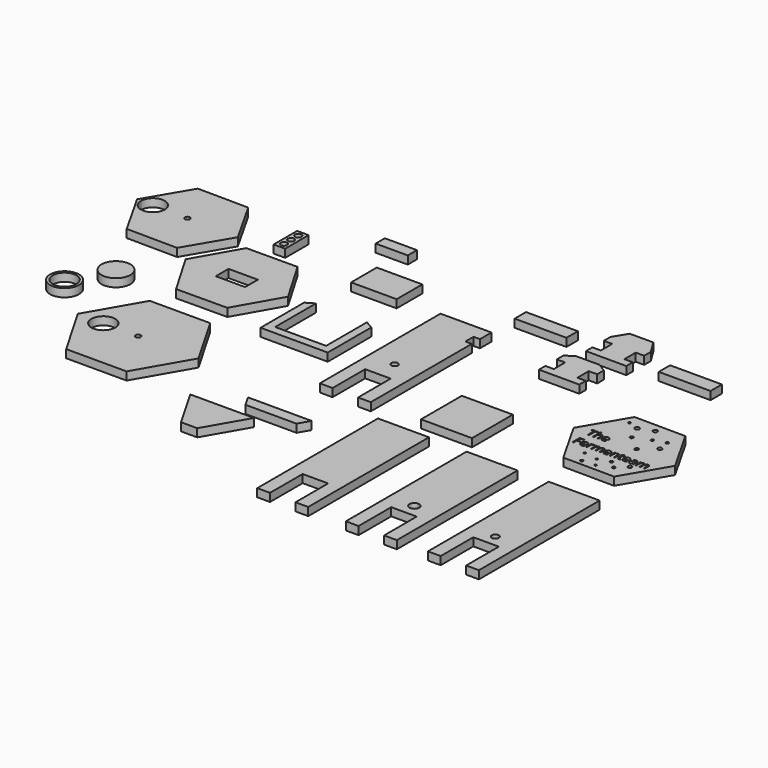
from build123d import *

# Parameters (mm, degrees)
F0_W     = 23
F0_H     = 12.5
F1_DEPTH = 6.35
F0_R     = 11.32
F0_W_2   = 40.64
F0_H_2   = 11.1560076475
F0_W_3   = 5
F0_H_3   = 11.35
F0_R_2   = 9.32
F0_R_3   = 1.1414075771
F0_R_4   = 0.7749819398
F0_R_5   = 0.8220081557
F0_R_6   = 0.8376599841
F0_R_7   = 1.1188046282
F0_R_8   = 1.1999997968
F0_R_9   = 1.5179013783
F0_R_10  = 1.4137050081
F0_R_11  = 1.2987416609
F0_R_12  = 1.1020189368
F0_R_13  = 0.9293109179
F0_R_14  = 1.7424434423
F0_R_15  = 1.6632093964
F0_R_16  = 1.1616311967
F0_R_17  = 1.6631997695
F0_W_4   = 25.2
F0_H_4   = 9
F0_W_5   = 15
F0_H_5   = 40
F0_W_6   = 10
F0_W_7   = 35.7
F0_H_6   = 25.2


# Not quite as in the source:
# - a feature names something its author has since deleted; it is built from what else it names


with BuildPart() as f1:
    # F0 (on Top) → F1 (new body)
    with BuildSketch(Plane.XY):
        Polygon((-93.5948539071, 0.11056655), (-73.7855066292, 34.8609587841), (-93.9755554565, 69.3915528762), (-133.9749515616, 69.1717547342), (-153.7842988395, 34.4213625001), (-133.5942500122, -0.109231592), align=None)
        with Locations((-113.7849027343, 34.6411606421)):
            Rectangle(F0_W, F0_H, mode=Mode.SUBTRACT)
    extrude(amount=F1_DEPTH)


with BuildPart() as f1b:
    # F0 (on Top) → F1, piece 2 (new body)
    with BuildSketch(Plane.XY):
        with Locations((-178.4373819828, -2.9960221145)):
            Circle(F0_R)
    extrude(amount=F1_DEPTH)


with BuildPart() as f1c:
    # F0 (on Top) → F1, piece 3 (new body)
    with BuildSketch(Plane.XY):
        Polygon((-20.9351536468, -136.0760015618), (-8.2351536468, -136.0760015618), (10.4148463532, -103.7732540007), (-39.5851536468, -103.7732540007), align=None)
    extrude(amount=F1_DEPTH)


with BuildPart() as f1d:
    # F0 (on Top) → F1, piece 4 (new body)
    with BuildSketch(Plane.XY):
        Polygon((40.420912765, -84.742741209), (-9.579087235, -84.742741209), (-4.579087235, -93.4029952469), (35.420912765, -93.4029952469), align=None)
    extrude(amount=F1_DEPTH)


with BuildPart() as f1e:
    # F0 (on Top) → F1, piece 5 (new body)
    with BuildSketch(Plane.XY):
        Polygon((138.8155827246, 127.2342521906), (120.3497827246, 127.2342521906), (113.7457827246, 116.4570544124), (113.7457827246, 109.9662874103), (120.3497827246, 109.9662874103), (120.3497827246, 98.8102797627), (113.7457827246, 98.8102797627), (113.7457827246, 92.4602797627), (145.4195827246, 92.4602797627), (145.4195827246, 98.8102797627), (138.8155827246, 98.8102797627), (138.8155827246, 109.9662874103), (145.4195827246, 109.9662874103), (145.4195827246, 116.4570544124), align=None)
    extrude(amount=F1_DEPTH)


with BuildPart() as f1f:
    # F0 (on Top) → F1, piece 6 (new body)
    with BuildSketch(Plane.XY):
        with Locations((186.0756911215, 104.3882835865)):
            Rectangle(F0_W_2, F0_H_2)
    extrude(amount=F1_DEPTH)


with BuildPart() as f1g:
    # F0 (on Top) → F1, piece 7 (new body)
    with BuildSketch(Plane.XY):
        with Locations((73.0896743277, 104.3882835865)):
            Rectangle(F0_W_2, F0_H_2)
    extrude(amount=F1_DEPTH)


with BuildPart() as f1h:
    # F0 (on Top) → F1, piece 8 (new body)
    with BuildSketch(Plane.XY):
        with BuildLine():
            Line((33.1884920597, 75.6191478133), (13.1884920597, 75.6191478133))
            Line((13.1884920597, 75.6191478133), (13.1884920597, -42.7308521867))
            Line((13.1884920597, -42.7308521867), (23.1884920597, -42.7308521867))
            Line((23.1884920597, -42.7308521867), (23.1884920597, -10.7308521867))
            Line((23.1884920597, -10.7308521867), (33.1884920597, -10.7308521867))
            Line((33.1884920597, -10.7308521867), (33.1884920597, 3.0191478133))
            ThreePointArc((33.1884920597, 3.0191478133), (30.5884920597, 5.6191478133), (33.1884920597, 8.2191478133))
            Line((33.1884920597, 8.2191478133), (33.1884920597, 75.6191478133))
        make_face()
        with BuildLine():
            Line((48.1884920597, 75.6191478133), (33.1884920597, 75.6191478133))
            Line((33.1884920597, 75.6191478133), (33.1884920597, 8.2191478133))
            ThreePointArc((33.1884920597, 8.2191478133), (35.0269696908, 7.4576254444), (35.7884920597, 5.6191478133))
            ThreePointArc((35.7884920597, 5.6191478133), (35.0269696908, 3.7806701822), (33.1884920597, 3.0191478133))
            Line((33.1884920597, 3.0191478133), (33.1884920597, -10.7308521867))
            Line((33.1884920597, -10.7308521867), (43.1884920597, -10.7308521867))
            Line((43.1884920597, -10.7308521867), (43.1884920597, -42.7308521867))
            Line((43.1884920597, -42.7308521867), (53.1884920597, -42.7308521867))
            Line((53.1884920597, -42.7308521867), (53.1884920597, 56.2691478133))
            Line((53.1884920597, 56.2691478133), (48.1884920597, 56.2691478133))
            Line((48.1884920597, 56.2691478133), (48.1884920597, 64.2691478133))
            Line((48.1884920597, 64.2691478133), (48.1884920597, 75.6191478133))
        make_face()
        with Locations((50.6884920597, 69.9441478133)):
            Rectangle(F0_W_3, F0_H_3)
    extrude(amount=F1_DEPTH)


with BuildPart() as f1i:
    # F0 (on Top) → F1, piece 9 (new body)
    with BuildSketch(Plane.XY):
        with Locations((-194.700971096, -33.0629588499)):
            Circle(F0_R)
        with Locations((-194.700971096, -33.0629588499)):
            Circle(F0_R_2, mode=Mode.SUBTRACT)
    extrude(amount=F1_DEPTH)


with BuildPart() as f1j:
    # F0 (on Top) → F1, piece 10 (new body)
    with BuildSketch(Plane.XY):
        Polygon((-136.4517834177, -104.2957006316), (-89.1217834177, -104.2957006316), (-65.4567834177, -63.3067182704), (-89.1217834177, -22.3177359093), (-136.4517834177, -22.3177359093), (-160.1167834177, -63.3067182704), align=None)
        with BuildLine():
            ThreePointArc((-130.7867834177, -63.3067182704), (-140.1067834177, -72.6267182704), (-149.4267834177, -63.3067182704))
            ThreePointArc((-149.4267834177, -63.3067182704), (-140.1067834177, -53.9867182704), (-130.7867834177, -63.3067182704))
        make_face(mode=Mode.SUBTRACT)
        with BuildLine():
            ThreePointArc((-110.7867834177, -63.3067182704), (-112.7867834177, -65.3067182704), (-114.7867834177, -63.3067182704))
            ThreePointArc((-114.7867834177, -63.3067182704), (-112.7867834177, -61.3067182704), (-110.7867834177, -63.3067182704))
        make_face(mode=Mode.SUBTRACT)
    extrude(amount=F1_DEPTH)


with BuildPart() as f1k:
    # F0 (on Top) → F1, piece 11 (new body)
    with BuildSketch(Plane.XY):
        Polygon((-207.0955206407, 43.3388591181), (-167.2973292077, 42.9594402712), (-147.0696471311, 77.2359756534), (-166.6401564875, 111.8919298825), (-206.4383479205, 112.2713487294), (-226.6660299971, 77.9948133472), align=None)
        with BuildLine():
            ThreePointArc((-204.8670206192, 77.7869909637), (-214.2754459411, 68.5562633129), (-223.5061735919, 77.9646886347))
            ThreePointArc((-223.5061735919, 77.9646886347), (-214.1421721831, 87.1957339202), (-204.8665971055, 77.8758397992))
            ThreePointArc((-204.8665971055, 77.8758397992), (-204.8667029846, 77.8314148768), (-204.8670206192, 77.7869909637))
        make_face(mode=Mode.SUBTRACT)
        with BuildLine():
            ThreePointArc((-184.8678385641, 77.6153945003), (-186.8773718092, 75.6154172211), (-188.8677476813, 77.634460774))
            ThreePointArc((-188.8677476813, 77.634460774), (-186.8583053189, 79.6153717795), (-184.8678385641, 77.6153945003))
        make_face(mode=Mode.SUBTRACT)
    extrude(amount=F1_DEPTH)


with BuildPart() as f1l:
    # F0 (on Top) → F1, piece 12 (new body)
    with BuildSketch(Plane.XY):
        Polygon((251.4182813621, 7.740817484), (231.6635930538, 42.5234644066), (191.6635930538, 42.806725949), (171.4182813621, 8.3073405689), (191.1729696704, -26.4753063537), (231.1729696704, -26.7585678962), align=None)
        with Locations((202.5459110737, -22.6449556649)):
            Circle(F0_R_3, mode=Mode.SUBTRACT)
        with Locations((212.8806561232, -22.0124032348)):
            Circle(F0_R_4, mode=Mode.SUBTRACT)
        Polygon((183.5228956864, -3.8237476475), (183.5228956864, -6.7932858103), (182.7155097343, -6.7932858103), (182.7155097343, 0.1538825798), (186.5882254029, 0.1538825798), (186.5882254029, -0.563793822), (183.5228956864, -0.563793822), (183.5228956864, -3.1060712456), (186.402724299, -3.1060712456), (186.402724299, -3.8237476475), align=None, mode=Mode.SUBTRACT)
        with BuildLine():
            add(Edge.make_bspline(
                [(190.7194262162, -6.8100113196), (190.3469035076, -6.8890773639), (189.8192897122, -6.8890773639)],
                knots=[0, 0, 0, 1, 1, 1], degree=2))
            add(Edge.make_bspline(
                [(189.8192897122, -6.8890773639), (188.6652295659, -6.8890773639), (187.9969694417, -6.1850854697)],
                knots=[0, 0, 0, 1, 1, 1], degree=2))
            add(Edge.make_bspline(
                [(187.9969694417, -6.1850854697), (187.3287093175, -5.4810935755), (187.3287093175, -4.2327623765)],
                knots=[0, 0, 0, 1, 1, 1], degree=2))
            add(Edge.make_bspline(
                [(187.3287093175, -4.2327623765), (187.3287093175, -2.9722671707), (187.9490736649, -2.2310230056)],
                knots=[0, 0, 0, 1, 1, 1], degree=2))
            add(Edge.make_bspline(
                [(187.9490736649, -2.2310230056), (188.5694380123, -1.4897788405), (189.6155425981, -1.4897788405)],
                knots=[0, 0, 0, 1, 1, 1], degree=2))
            add(Edge.make_bspline(
                [(189.6155425981, -1.4897788405), (190.5932246455, -1.4897788405), (191.1634124648, -2.1337109511)],
                knots=[0, 0, 0, 1, 1, 1], degree=2))
            add(Edge.make_bspline(
                [(191.1634124648, -2.1337109511), (191.7336002841, -2.7776430617), (191.7336002841, -3.8328706526)],
                knots=[0, 0, 0, 1, 1, 1], degree=2))
            Line((191.7336002841, -3.8328706526), (191.7336002841, -4.3315949318))
            Line((191.7336002841, -4.3315949318), (188.1467387756, -4.3315949318))
            add(Edge.make_bspline(
                [(188.1467387756, -4.3315949318), (188.1710667892, -5.2484569452), (188.6104915353, -5.7236134613)],
                knots=[0, 0, 0, 1, 1, 1], degree=2))
            add(Edge.make_bspline(
                [(188.6104915353, -5.7236134613), (189.0499162813, -6.1987699774), (189.8481792283, -6.1987699774)],
                knots=[0, 0, 0, 1, 1, 1], degree=2))
            add(Edge.make_bspline(
                [(189.8481792283, -6.1987699774), (190.6890161992, -6.1987699774), (191.5100866589, -5.8475342807)],
                knots=[0, 0, 0, 1, 1, 1], degree=2))
            Line((191.5100866589, -5.8475342807), (191.5100866589, -6.5515261749))
            add(Edge.make_bspline(
                [(191.5100866589, -6.5515261749), (191.0919489248, -6.7309452754), (190.7194262162, -6.8100113196)],
                knots=[0, 0, 0, 1, 1, 1], degree=2))
        make_face(mode=Mode.SUBTRACT)
        Polygon((184.8533339314, 12.6706455887), (184.8533339314, 6.4411536005), (184.0459479793, 6.4411536005), (184.0459479793, 12.6706455887), (181.8457832473, 12.6706455887), (181.8457832473, 13.3883219906), (187.0534986634, 13.3883219906), (187.0534986634, 12.6706455887), align=None, mode=Mode.SUBTRACT)
        with BuildLine():
            Line((192.3341981204, 6.4411536005), (191.5450581785, 6.4411536005))
            Line((191.5450581785, 6.4411536005), (191.5450581785, 9.8105834872))
            add(Edge.make_bspline(
                [(191.5450581785, 9.8105834872), (191.5450581785, 10.4461528431), (191.2554027663, 10.7601362689)],
                knots=[0, 0, 0, 1, 1, 1], degree=2))
            add(Edge.make_bspline(
                [(191.2554027663, 10.7601362689), (190.9657473541, 11.0741196947), (190.3469035076, 11.0741196947)],
                knots=[0, 0, 0, 1, 1, 1], degree=2))
            add(Edge.make_bspline(
                [(190.3469035076, 11.0741196947), (189.5258330478, 11.0741196947), (189.1479885863, 10.6270924444)],
                knots=[0, 0, 0, 1, 1, 1], degree=2))
            add(Edge.make_bspline(
                [(189.1479885863, 10.6270924444), (188.7701441247, 10.1800651941), (188.7701441247, 9.1643706253)],
                knots=[0, 0, 0, 1, 1, 1], degree=2))
            Line((188.7701441247, 9.1643706253), (188.7701441247, 6.4411536005))
            Line((188.7701441247, 6.4411536005), (187.9810041828, 6.4411536005))
            Line((187.9810041828, 6.4411536005), (187.9810041828, 13.8353492409))
            Line((187.9810041828, 13.8353492409), (188.7701441247, 13.8353492409))
            Line((188.7701441247, 13.8353492409), (188.7701441247, 11.5971719876))
            add(Edge.make_bspline(
                [(188.7701441247, 11.5971719876), (188.7701441247, 11.1927187611), (188.7321316034, 10.9266311121)],
                knots=[0, 0, 0, 1, 1, 1], degree=2))
            Line((188.7321316034, 10.9266311121), (188.7792671298, 10.9266311121))
            add(Edge.make_bspline(
                [(188.7792671298, 10.9266311121), (189.01190376, 11.3021948224), (189.442205501, 11.5181059433)],
                knots=[0, 0, 0, 1, 1, 1], degree=2))
            add(Edge.make_bspline(
                [(189.442205501, 11.5181059433), (189.872507242, 11.7340170642), (190.4229285502, 11.7340170642)],
                knots=[0, 0, 0, 1, 1, 1], degree=2))
            add(Edge.make_bspline(
                [(190.4229285502, 11.7340170642), (191.3778030849, 11.7340170642), (191.8560006026, 11.2801475601)],
                knots=[0, 0, 0, 1, 1, 1], degree=2))
            add(Edge.make_bspline(
                [(191.8560006026, 11.2801475601), (192.3341981204, 10.8262780559), (192.3341981204, 9.8379525025)],
                knots=[0, 0, 0, 1, 1, 1], degree=2))
            Line((192.3341981204, 9.8379525025), (192.3341981204, 6.4411536005))
        make_face(mode=Mode.SUBTRACT)
        with Locations((197.5992619991, -13.4883988649)):
            Circle(F0_R_5, mode=Mode.SUBTRACT)
        with Locations((208.3211392164, -15.1996426284)):
            Circle(F0_R_6, mode=Mode.SUBTRACT)
        with Locations((217.7015841007, -12.4359205365)):
            Circle(F0_R_7, mode=Mode.SUBTRACT)
        with BuildLine():
            add(Edge.make_bspline(
                [(194.5571703652, -1.7657497451), (194.9661850942, -1.4897788405), (195.4557863684, -1.4897788405)],
                knots=[0, 0, 0, 1, 1, 1], degree=2))
            add(Edge.make_bspline(
                [(195.4557863684, -1.4897788405), (195.8024605625, -1.4897788405), (196.0776712166, -1.5475578729)],
                knots=[0, 0, 0, 1, 1, 1], degree=2))
            Line((196.0776712166, -1.5475578729), (195.9681951553, -2.2789187824))
            add(Edge.make_bspline(
                [(195.9681951553, -2.2789187824), (195.6458489748, -2.2074552424), (195.398007336, -2.2074552424)],
                knots=[0, 0, 0, 1, 1, 1], degree=2))
            add(Edge.make_bspline(
                [(195.398007336, -2.2074552424), (194.7654789818, -2.2074552424), (194.3169312306, -2.7206242798)],
                knots=[0, 0, 0, 1, 1, 1], degree=2))
            add(Edge.make_bspline(
                [(194.3169312306, -2.7206242798), (193.8683834795, -3.2337933171), (193.8683834795, -3.9986052454)],
                knots=[0, 0, 0, 1, 1, 1], degree=2))
            Line((193.8683834795, -3.9986052454), (193.8683834795, -6.7932858103))
            Line((193.8683834795, -6.7932858103), (193.0792435376, -6.7932858103))
            Line((193.0792435376, -6.7932858103), (193.0792435376, -1.5855703942))
            Line((193.0792435376, -1.5855703942), (193.730017902, -1.5855703942))
            Line((193.730017902, -1.5855703942), (193.8212479531, -2.549567934))
            Line((193.8212479531, -2.549567934), (193.8592604744, -2.549567934))
            add(Edge.make_bspline(
                [(193.8592604744, -2.549567934), (194.1481556361, -2.0417206496), (194.5571703652, -1.7657497451)],
                knots=[0, 0, 0, 1, 1, 1], degree=2))
        make_face(mode=Mode.SUBTRACT)
        with BuildLine():
            Line((204.4784384207, -6.7932858103), (203.6908189796, -6.7932858103))
            Line((203.6908189796, -6.7932858103), (203.6908189796, -3.4056099133))
            add(Edge.make_bspline(
                [(203.6908189796, -3.4056099133), (203.6908189796, -2.7822045642), (203.4247313306, -2.4712621401)],
                knots=[0, 0, 0, 1, 1, 1], degree=2))
            add(Edge.make_bspline(
                [(203.4247313306, -2.4712621401), (203.1586436816, -2.160319716), (202.5975788675, -2.160319716)],
                knots=[0, 0, 0, 1, 1, 1], degree=2))
            add(Edge.make_bspline(
                [(202.5975788675, -2.160319716), (201.8616564554, -2.160319716), (201.5096605083, -2.5830189527)],
                knots=[0, 0, 0, 1, 1, 1], degree=2))
            add(Edge.make_bspline(
                [(201.5096605083, -2.5830189527), (201.1576645612, -3.0057181894), (201.1576645612, -3.8845676815)],
                knots=[0, 0, 0, 1, 1, 1], degree=2))
            Line((201.1576645612, -3.8845676815), (201.1576645612, -6.7932858103))
            Line((201.1576645612, -6.7932858103), (200.3685246193, -6.7932858103))
            Line((200.3685246193, -6.7932858103), (200.3685246193, -3.4056099133))
            add(Edge.make_bspline(
                [(200.3685246193, -3.4056099133), (200.3685246193, -2.7822045642), (200.1024369703, -2.4712621401)],
                knots=[0, 0, 0, 1, 1, 1], degree=2))
            add(Edge.make_bspline(
                [(200.1024369703, -2.4712621401), (199.8363493213, -2.160319716), (199.2707230046, -2.160319716)],
                knots=[0, 0, 0, 1, 1, 1], degree=2))
            add(Edge.make_bspline(
                [(199.2707230046, -2.160319716), (198.5302390899, -2.160319716), (198.1858456471, -2.6043059646)],
                knots=[0, 0, 0, 1, 1, 1], degree=2))
            add(Edge.make_bspline(
                [(198.1858456471, -2.6043059646), (197.8414522042, -3.0482922132), (197.8414522042, -4.0609457803)],
                knots=[0, 0, 0, 1, 1, 1], degree=2))
            Line((197.8414522042, -4.0609457803), (197.8414522042, -6.7932858103))
            Line((197.8414522042, -6.7932858103), (197.0523122623, -6.7932858103))
            Line((197.0523122623, -6.7932858103), (197.0523122623, -1.5855703942))
            Line((197.0523122623, -1.5855703942), (197.6939636216, -1.5855703942))
            Line((197.6939636216, -1.5855703942), (197.8216856932, -2.2986852935))
            Line((197.8216856932, -2.2986852935), (197.8596982144, -2.2986852935))
            add(Edge.make_bspline(
                [(197.8596982144, -2.2986852935), (198.0832118396, -1.9185600806), (198.4899458174, -1.7041694606)],
                knots=[0, 0, 0, 1, 1, 1], degree=2))
            add(Edge.make_bspline(
                [(198.4899458174, -1.7041694606), (198.8966797951, -1.4897788405), (199.3999655769, -1.4897788405)],
                knots=[0, 0, 0, 1, 1, 1], degree=2))
            add(Edge.make_bspline(
                [(199.3999655769, -1.4897788405), (200.6209277606, -1.4897788405), (200.9964914709, -2.3747103361)],
                knots=[0, 0, 0, 1, 1, 1], degree=2))
            Line((200.9964914709, -2.3747103361), (201.0345039922, -2.3747103361))
            add(Edge.make_bspline(
                [(201.0345039922, -2.3747103361), (201.2671406225, -1.965695607), (201.7088461198, -1.7277372238)],
                knots=[0, 0, 0, 1, 1, 1], degree=2))
            add(Edge.make_bspline(
                [(201.7088461198, -1.7277372238), (202.1505516171, -1.4897788405), (202.7161779339, -1.4897788405)],
                knots=[0, 0, 0, 1, 1, 1], degree=2))
            add(Edge.make_bspline(
                [(202.7161779339, -1.4897788405), (203.5995889285, -1.4897788405), (204.0390136746, -1.9436483447)],
                knots=[0, 0, 0, 1, 1, 1], degree=2))
            add(Edge.make_bspline(
                [(204.0390136746, -1.9436483447), (204.4784384207, -2.3975178488), (204.4784384207, -3.3964869082)],
                knots=[0, 0, 0, 1, 1, 1], degree=2))
            Line((204.4784384207, -3.3964869082), (204.4784384207, -6.7932858103))
        make_face(mode=Mode.SUBTRACT)
        with BuildLine():
            add(Edge.make_bspline(
                [(209.2041550669, -6.8100113196), (208.8316323583, -6.8890773639), (208.3040185628, -6.8890773639)],
                knots=[0, 0, 0, 1, 1, 1], degree=2))
            add(Edge.make_bspline(
                [(208.3040185628, -6.8890773639), (207.1499584166, -6.8890773639), (206.4816982924, -6.1850854697)],
                knots=[0, 0, 0, 1, 1, 1], degree=2))
            add(Edge.make_bspline(
                [(206.4816982924, -6.1850854697), (205.8134381682, -5.4810935755), (205.8134381682, -4.2327623765)],
                knots=[0, 0, 0, 1, 1, 1], degree=2))
            add(Edge.make_bspline(
                [(205.8134381682, -4.2327623765), (205.8134381682, -2.9722671707), (206.4338025156, -2.2310230056)],
                knots=[0, 0, 0, 1, 1, 1], degree=2))
            add(Edge.make_bspline(
                [(206.4338025156, -2.2310230056), (207.054166863, -1.4897788405), (208.1002714487, -1.4897788405)],
                knots=[0, 0, 0, 1, 1, 1], degree=2))
            add(Edge.make_bspline(
                [(208.1002714487, -1.4897788405), (209.0779534962, -1.4897788405), (209.6481413155, -2.1337109511)],
                knots=[0, 0, 0, 1, 1, 1], degree=2))
            add(Edge.make_bspline(
                [(209.6481413155, -2.1337109511), (210.2183291348, -2.7776430617), (210.2183291348, -3.8328706526)],
                knots=[0, 0, 0, 1, 1, 1], degree=2))
            Line((210.2183291348, -3.8328706526), (210.2183291348, -4.3315949318))
            Line((210.2183291348, -4.3315949318), (206.6314676263, -4.3315949318))
            add(Edge.make_bspline(
                [(206.6314676263, -4.3315949318), (206.6557956399, -5.2484569452), (207.095220386, -5.7236134613)],
                knots=[0, 0, 0, 1, 1, 1], degree=2))
            add(Edge.make_bspline(
                [(207.095220386, -5.7236134613), (207.534645132, -6.1987699774), (208.332908079, -6.1987699774)],
                knots=[0, 0, 0, 1, 1, 1], degree=2))
            add(Edge.make_bspline(
                [(208.332908079, -6.1987699774), (209.1737450498, -6.1987699774), (209.9948155096, -5.8475342807)],
                knots=[0, 0, 0, 1, 1, 1], degree=2))
            Line((209.9948155096, -5.8475342807), (209.9948155096, -6.5515261749))
            add(Edge.make_bspline(
                [(209.9948155096, -6.5515261749), (209.5766777755, -6.7309452754), (209.2041550669, -6.8100113196)],
                knots=[0, 0, 0, 1, 1, 1], degree=2))
        make_face(mode=Mode.SUBTRACT)
        with BuildLine():
            Line((215.9171663259, -6.7932858103), (215.128026384, -6.7932858103))
            Line((215.128026384, -6.7932858103), (215.128026384, -3.4238559235))
            add(Edge.make_bspline(
                [(215.128026384, -3.4238559235), (215.128026384, -2.7882865676), (214.8383709718, -2.4743031418)],
                knots=[0, 0, 0, 1, 1, 1], degree=2))
            add(Edge.make_bspline(
                [(214.8383709718, -2.4743031418), (214.5487155596, -2.160319716), (213.9298717131, -2.160319716)],
                knots=[0, 0, 0, 1, 1, 1], degree=2))
            add(Edge.make_bspline(
                [(213.9298717131, -2.160319716), (213.1133627559, -2.160319716), (212.733237543, -2.6020252133)],
                knots=[0, 0, 0, 1, 1, 1], degree=2))
            add(Edge.make_bspline(
                [(212.733237543, -2.6020252133), (212.3531123302, -3.0437307107), (212.3531123302, -4.0609457803)],
                knots=[0, 0, 0, 1, 1, 1], degree=2))
            Line((212.3531123302, -4.0609457803), (212.3531123302, -6.7932858103))
            Line((212.3531123302, -6.7932858103), (211.5639723883, -6.7932858103))
            Line((211.5639723883, -6.7932858103), (211.5639723883, -1.5855703942))
            Line((211.5639723883, -1.5855703942), (212.2056237476, -1.5855703942))
            Line((212.2056237476, -1.5855703942), (212.3333458191, -2.2986852935))
            Line((212.3333458191, -2.2986852935), (212.3713583404, -2.2986852935))
            add(Edge.make_bspline(
                [(212.3713583404, -2.2986852935), (212.6146384766, -1.9139985781), (213.0517824714, -1.7018887093)],
                knots=[0, 0, 0, 1, 1, 1], degree=2))
            add(Edge.make_bspline(
                [(213.0517824714, -1.7018887093), (213.4889264662, -1.4897788405), (214.0256632667, -1.4897788405)],
                knots=[0, 0, 0, 1, 1, 1], degree=2))
            add(Edge.make_bspline(
                [(214.0256632667, -1.4897788405), (214.9668532937, -1.4897788405), (215.4420098098, -1.9436483447)],
                knots=[0, 0, 0, 1, 1, 1], degree=2))
            add(Edge.make_bspline(
                [(215.4420098098, -1.9436483447), (215.9171663259, -2.3975178488), (215.9171663259, -3.3964869082)],
                knots=[0, 0, 0, 1, 1, 1], degree=2))
            Line((215.9171663259, -3.3964869082), (215.9171663259, -6.7932858103))
        make_face(mode=Mode.SUBTRACT)
        with BuildLine():
            add(Edge.make_bspline(
                [(218.6054118312, -5.9851396078), (218.8289254563, -6.2367824987), (219.2181736743, -6.2367824987)],
                knots=[0, 0, 0, 1, 1, 1], degree=2))
            add(Edge.make_bspline(
                [(219.2181736743, -6.2367824987), (219.4280027918, -6.2367824987), (219.6226269008, -6.2063724816)],
                knots=[0, 0, 0, 1, 1, 1], degree=2))
            add(Edge.make_bspline(
                [(219.6226269008, -6.2063724816), (219.8172510098, -6.1759624646), (219.9312885736, -6.1425114459)],
                knots=[0, 0, 0, 1, 1, 1], degree=2))
            Line((219.9312885736, -6.1425114459), (219.9312885736, -6.7461502839))
            add(Edge.make_bspline(
                [(219.9312885736, -6.7461502839), (219.8035665021, -6.8069703179), (219.5542043625, -6.8480238409)],
                knots=[0, 0, 0, 1, 1, 1], degree=2))
            add(Edge.make_bspline(
                [(219.5542043625, -6.8480238409), (219.3048422228, -6.8890773639), (219.1041361105, -6.8890773639)],
                knots=[0, 0, 0, 1, 1, 1], degree=2))
            add(Edge.make_bspline(
                [(219.1041361105, -6.8890773639), (217.594278765, -6.8890773639), (217.594278765, -5.2971129725)],
                knots=[0, 0, 0, 1, 1, 1], degree=2))
            Line((217.594278765, -5.2971129725), (217.594278765, -2.1983322373))
            Line((217.594278765, -2.1983322373), (216.847712847, -2.1983322373))
            Line((216.847712847, -2.1983322373), (216.847712847, -1.8182070244))
            Line((216.847712847, -1.8182070244), (217.594278765, -1.4897788405))
            Line((217.594278765, -1.4897788405), (217.9257479506, -0.3782927181))
            Line((217.9257479506, -0.3782927181), (218.381898206, -0.3782927181))
            Line((218.381898206, -0.3782927181), (218.381898206, -1.5855703942))
            Line((218.381898206, -1.5855703942), (219.8932760523, -1.5855703942))
            Line((219.8932760523, -1.5855703942), (219.8932760523, -2.1983322373))
            Line((219.8932760523, -2.1983322373), (218.381898206, -2.1983322373))
            Line((218.381898206, -2.1983322373), (218.381898206, -5.2636619538))
            add(Edge.make_bspline(
                [(218.381898206, -5.2636619538), (218.381898206, -5.7334967168), (218.6054118312, -5.9851396078)],
                knots=[0, 0, 0, 1, 1, 1], degree=2))
        make_face(mode=Mode.SUBTRACT)
        with Locations((223.384976387, -17.3825658858)):
            Circle(F0_R_8, mode=Mode.SUBTRACT)
        with Locations((230.6536883116, -10.4995090514)):
            Circle(F0_R_9, mode=Mode.SUBTRACT)
        with BuildLine():
            add(Edge.make_bspline(
                [(224.071612392, -6.8100113196), (223.6990896834, -6.8890773639), (223.171475888, -6.8890773639)],
                knots=[0, 0, 0, 1, 1, 1], degree=2))
            add(Edge.make_bspline(
                [(223.171475888, -6.8890773639), (222.0174157418, -6.8890773639), (221.3491556176, -6.1850854697)],
                knots=[0, 0, 0, 1, 1, 1], degree=2))
            add(Edge.make_bspline(
                [(221.3491556176, -6.1850854697), (220.6808954934, -5.4810935755), (220.6808954934, -4.2327623765)],
                knots=[0, 0, 0, 1, 1, 1], degree=2))
            add(Edge.make_bspline(
                [(220.6808954934, -4.2327623765), (220.6808954934, -2.9722671707), (221.3012598408, -2.2310230056)],
                knots=[0, 0, 0, 1, 1, 1], degree=2))
            add(Edge.make_bspline(
                [(221.3012598408, -2.2310230056), (221.9216241881, -1.4897788405), (222.9677287739, -1.4897788405)],
                knots=[0, 0, 0, 1, 1, 1], degree=2))
            add(Edge.make_bspline(
                [(222.9677287739, -1.4897788405), (223.9454108214, -1.4897788405), (224.5155986407, -2.1337109511)],
                knots=[0, 0, 0, 1, 1, 1], degree=2))
            add(Edge.make_bspline(
                [(224.5155986407, -2.1337109511), (225.0857864599, -2.7776430617), (225.0857864599, -3.8328706526)],
                knots=[0, 0, 0, 1, 1, 1], degree=2))
            Line((225.0857864599, -3.8328706526), (225.0857864599, -4.3315949318))
            Line((225.0857864599, -4.3315949318), (221.4989249514, -4.3315949318))
            add(Edge.make_bspline(
                [(221.4989249514, -4.3315949318), (221.5232529651, -5.2484569452), (221.9626777111, -5.7236134613)],
                knots=[0, 0, 0, 1, 1, 1], degree=2))
            add(Edge.make_bspline(
                [(221.9626777111, -5.7236134613), (222.4021024572, -6.1987699774), (223.2003654042, -6.1987699774)],
                knots=[0, 0, 0, 1, 1, 1], degree=2))
            add(Edge.make_bspline(
                [(223.2003654042, -6.1987699774), (224.041202375, -6.1987699774), (224.8622728348, -5.8475342807)],
                knots=[0, 0, 0, 1, 1, 1], degree=2))
            Line((224.8622728348, -5.8475342807), (224.8622728348, -6.5515261749))
            add(Edge.make_bspline(
                [(224.8622728348, -6.5515261749), (224.4441351006, -6.7309452754), (224.071612392, -6.8100113196)],
                knots=[0, 0, 0, 1, 1, 1], degree=2))
        make_face(mode=Mode.SUBTRACT)
        with BuildLine():
            Line((230.2189973343, -6.7932858103), (229.6336045065, -6.7932858103))
            Line((229.6336045065, -6.7932858103), (229.4769929188, -6.0512813948))
            Line((229.4769929188, -6.0512813948), (229.4389803975, -6.0512813948))
            add(Edge.make_bspline(
                [(229.4389803975, -6.0512813948), (229.0497321796, -6.5408826689), (228.6627647129, -6.7149800164)],
                knots=[0, 0, 0, 1, 1, 1], degree=2))
            add(Edge.make_bspline(
                [(228.6627647129, -6.7149800164), (228.2757972462, -6.8890773639), (227.694965921, -6.8890773639)],
                knots=[0, 0, 0, 1, 1, 1], degree=2))
            add(Edge.make_bspline(
                [(227.694965921, -6.8890773639), (226.9210309876, -6.8890773639), (226.4816062415, -6.48918564)],
                knots=[0, 0, 0, 1, 1, 1], degree=2))
            add(Edge.make_bspline(
                [(226.4816062415, -6.48918564), (226.0421814955, -6.0892939161), (226.0421814955, -5.353371504)],
                knots=[0, 0, 0, 1, 1, 1], degree=2))
            add(Edge.make_bspline(
                [(226.0421814955, -5.353371504), (226.0421814955, -3.7766121211), (228.564692408, -3.7005870785)],
                knots=[0, 0, 0, 1, 1, 1], degree=2))
            Line((228.564692408, -3.7005870785), (229.4481034026, -3.6716975623))
            Line((229.4481034026, -3.6716975623), (229.4481034026, -3.347830881))
            add(Edge.make_bspline(
                [(229.4481034026, -3.347830881), (229.4481034026, -2.7350690378), (229.1850567554, -2.4431328744)],
                knots=[0, 0, 0, 1, 1, 1], degree=2))
            add(Edge.make_bspline(
                [(229.1850567554, -2.4431328744), (228.9220101081, -2.1511967109), (228.3411787828, -2.1511967109)],
                knots=[0, 0, 0, 1, 1, 1], degree=2))
            add(Edge.make_bspline(
                [(228.3411787828, -2.1511967109), (227.6904044184, -2.1511967109), (226.8693339586, -2.549567934)],
                knots=[0, 0, 0, 1, 1, 1], degree=2))
            Line((226.8693339586, -2.549567934), (226.6260538224, -1.945929096))
            add(Edge.make_bspline(
                [(226.6260538224, -1.945929096), (227.0107405378, -1.7376204793), (227.4691715445, -1.6190214129)],
                knots=[0, 0, 0, 1, 1, 1], degree=2))
            add(Edge.make_bspline(
                [(227.4691715445, -1.6190214129), (227.9276025512, -1.5004223465), (228.3898348101, -1.5004223465)],
                knots=[0, 0, 0, 1, 1, 1], degree=2))
            add(Edge.make_bspline(
                [(228.3898348101, -1.5004223465), (229.3203813311, -1.5004223465), (229.7696893327, -1.9132383277)],
                knots=[0, 0, 0, 1, 1, 1], degree=2))
            add(Edge.make_bspline(
                [(229.7696893327, -1.9132383277), (230.2189973343, -2.3260543088), (230.2189973343, -3.2383548197)],
                knots=[0, 0, 0, 1, 1, 1], degree=2))
            Line((230.2189973343, -3.2383548197), (230.2189973343, -6.7932858103))
        make_face(mode=Mode.SUBTRACT)
        with BuildLine():
            Line((239.269018402, -6.7932858103), (238.4813989609, -6.7932858103))
            Line((238.4813989609, -6.7932858103), (238.4813989609, -3.4056099133))
            add(Edge.make_bspline(
                [(238.4813989609, -3.4056099133), (238.4813989609, -2.7822045642), (238.2153113119, -2.4712621401)],
                knots=[0, 0, 0, 1, 1, 1], degree=2))
            add(Edge.make_bspline(
                [(238.2153113119, -2.4712621401), (237.9492236629, -2.160319716), (237.3881588488, -2.160319716)],
                knots=[0, 0, 0, 1, 1, 1], degree=2))
            add(Edge.make_bspline(
                [(237.3881588488, -2.160319716), (236.6522364367, -2.160319716), (236.3002404896, -2.5830189527)],
                knots=[0, 0, 0, 1, 1, 1], degree=2))
            add(Edge.make_bspline(
                [(236.3002404896, -2.5830189527), (235.9482445425, -3.0057181894), (235.9482445425, -3.8845676815)],
                knots=[0, 0, 0, 1, 1, 1], degree=2))
            Line((235.9482445425, -3.8845676815), (235.9482445425, -6.7932858103))
            Line((235.9482445425, -6.7932858103), (235.1591046006, -6.7932858103))
            Line((235.1591046006, -6.7932858103), (235.1591046006, -3.4056099133))
            add(Edge.make_bspline(
                [(235.1591046006, -3.4056099133), (235.1591046006, -2.7822045642), (234.8930169516, -2.4712621401)],
                knots=[0, 0, 0, 1, 1, 1], degree=2))
            add(Edge.make_bspline(
                [(234.8930169516, -2.4712621401), (234.6269293026, -2.160319716), (234.0613029859, -2.160319716)],
                knots=[0, 0, 0, 1, 1, 1], degree=2))
            add(Edge.make_bspline(
                [(234.0613029859, -2.160319716), (233.3208190712, -2.160319716), (232.9764256284, -2.6043059646)],
                knots=[0, 0, 0, 1, 1, 1], degree=2))
            add(Edge.make_bspline(
                [(232.9764256284, -2.6043059646), (232.6320321855, -3.0482922132), (232.6320321855, -4.0609457803)],
                knots=[0, 0, 0, 1, 1, 1], degree=2))
            Line((232.6320321855, -4.0609457803), (232.6320321855, -6.7932858103))
            Line((232.6320321855, -6.7932858103), (231.8428922436, -6.7932858103))
            Line((231.8428922436, -6.7932858103), (231.8428922436, -1.5855703942))
            Line((231.8428922436, -1.5855703942), (232.4845436029, -1.5855703942))
            Line((232.4845436029, -1.5855703942), (232.6122656744, -2.2986852935))
            Line((232.6122656744, -2.2986852935), (232.6502781957, -2.2986852935))
            add(Edge.make_bspline(
                [(232.6502781957, -2.2986852935), (232.8737918209, -1.9185600806), (233.2805257986, -1.7041694606)],
                knots=[0, 0, 0, 1, 1, 1], degree=2))
            add(Edge.make_bspline(
                [(233.2805257986, -1.7041694606), (233.6872597764, -1.4897788405), (234.1905455582, -1.4897788405)],
                knots=[0, 0, 0, 1, 1, 1], degree=2))
            add(Edge.make_bspline(
                [(234.1905455582, -1.4897788405), (235.4115077419, -1.4897788405), (235.7870714522, -2.3747103361)],
                knots=[0, 0, 0, 1, 1, 1], degree=2))
            Line((235.7870714522, -2.3747103361), (235.8250839735, -2.3747103361))
            add(Edge.make_bspline(
                [(235.8250839735, -2.3747103361), (236.0577206038, -1.965695607), (236.4994261011, -1.7277372238)],
                knots=[0, 0, 0, 1, 1, 1], degree=2))
            add(Edge.make_bspline(
                [(236.4994261011, -1.7277372238), (236.9411315984, -1.4897788405), (237.5067579152, -1.4897788405)],
                knots=[0, 0, 0, 1, 1, 1], degree=2))
            add(Edge.make_bspline(
                [(237.5067579152, -1.4897788405), (238.3901689098, -1.4897788405), (238.8295936559, -1.9436483447)],
                knots=[0, 0, 0, 1, 1, 1], degree=2))
            add(Edge.make_bspline(
                [(238.8295936559, -1.9436483447), (239.269018402, -2.3975178488), (239.269018402, -3.3964869082)],
                knots=[0, 0, 0, 1, 1, 1], degree=2))
            Line((239.269018402, -3.3964869082), (239.269018402, -6.7932858103))
        make_face(mode=Mode.SUBTRACT)
        with BuildLine():
            add(Edge.make_bspline(
                [(197.0538327632, 6.4244280911), (196.6813100546, 6.3453620468), (196.1536962592, 6.3453620468)],
                knots=[0, 0, 0, 1, 1, 1], degree=2))
            add(Edge.make_bspline(
                [(196.1536962592, 6.3453620468), (194.9996361129, 6.3453620468), (194.3313759887, 7.049353941)],
                knots=[0, 0, 0, 1, 1, 1], degree=2))
            add(Edge.make_bspline(
                [(194.3313759887, 7.049353941), (193.6631158645, 7.7533458352), (193.6631158645, 9.0016770342)],
                knots=[0, 0, 0, 1, 1, 1], degree=2))
            add(Edge.make_bspline(
                [(193.6631158645, 9.0016770342), (193.6631158645, 10.2621722401), (194.2834802119, 11.0034164051)],
                knots=[0, 0, 0, 1, 1, 1], degree=2))
            add(Edge.make_bspline(
                [(194.2834802119, 11.0034164051), (194.9038445593, 11.7446605702), (195.9499491451, 11.7446605702)],
                knots=[0, 0, 0, 1, 1, 1], degree=2))
            add(Edge.make_bspline(
                [(195.9499491451, 11.7446605702), (196.9276311925, 11.7446605702), (197.4978190118, 11.1007284596)],
                knots=[0, 0, 0, 1, 1, 1], degree=2))
            add(Edge.make_bspline(
                [(197.4978190118, 11.1007284596), (198.0680068311, 10.4567963491), (198.0680068311, 9.4015687582)],
                knots=[0, 0, 0, 1, 1, 1], degree=2))
            Line((198.0680068311, 9.4015687582), (198.0680068311, 8.9028444789))
            Line((198.0680068311, 8.9028444789), (194.4811453226, 8.9028444789))
            add(Edge.make_bspline(
                [(194.4811453226, 8.9028444789), (194.5054733362, 7.9859824655), (194.9448980823, 7.5108259494)],
                knots=[0, 0, 0, 1, 1, 1], degree=2))
            add(Edge.make_bspline(
                [(194.9448980823, 7.5108259494), (195.3843228283, 7.0356694334), (196.1825857753, 7.0356694334)],
                knots=[0, 0, 0, 1, 1, 1], degree=2))
            add(Edge.make_bspline(
                [(196.1825857753, 7.0356694334), (197.0234227462, 7.0356694334), (197.8444932059, 7.38690513)],
                knots=[0, 0, 0, 1, 1, 1], degree=2))
            Line((197.8444932059, 7.38690513), (197.8444932059, 6.6829132358))
            add(Edge.make_bspline(
                [(197.8444932059, 6.6829132358), (197.4263554718, 6.5034941354), (197.0538327632, 6.4244280911)],
                knots=[0, 0, 0, 1, 1, 1], degree=2))
        make_face(mode=Mode.SUBTRACT)
        with Locations((219.2846983671, 10.2956565097)):
            Circle(F0_R_10, mode=Mode.SUBTRACT)
        with Locations((207.0433497429, 20.6947308034)):
            Circle(F0_R_11, mode=Mode.SUBTRACT)
        with Locations((219.3566262722, 25.5735795945)):
            Circle(F0_R_12, mode=Mode.SUBTRACT)
        with Locations((193.9169168472, 34.9827818573)):
            Circle(F0_R_13, mode=Mode.SUBTRACT)
        with Locations((202.2806555033, 32.0787094533)):
            Circle(F0_R_14, mode=Mode.SUBTRACT)
        with Locations((230.0436198711, 19.5331014693)):
            Circle(F0_R_15, mode=Mode.SUBTRACT)
        with Locations((228.6496609449, 28.5938177258)):
            Circle(F0_R_16, mode=Mode.SUBTRACT)
        with Locations((213.1999880075, 36.144413054)):
            Circle(F0_R_17, mode=Mode.SUBTRACT)
    extrude(amount=F1_DEPTH)


with BuildPart() as f1m:
    # F0 (on Top) → F1, piece 13 (new body)
    with BuildSketch(Plane.XY):
        with BuildLine():
            Line((-119.4307953119, 106.4602797627), (-123.9307953119, 106.4602797627))
            Line((-123.9307953119, 106.4602797627), (-123.9307953119, 83.4602797627))
            Line((-123.9307953119, 83.4602797627), (-119.4307953119, 83.4602797627))
            Line((-119.4307953119, 83.4602797627), (-119.4307953119, 85.4602797627))
            ThreePointArc((-119.4307953119, 85.4602797627), (-121.9307953119, 87.9602797627), (-119.4307953119, 90.4602797627))
            Line((-119.4307953119, 90.4602797627), (-119.4307953119, 92.4602797627))
            ThreePointArc((-119.4307953119, 92.4602797627), (-121.9307953119, 94.9602797627), (-119.4307953119, 97.4602797627))
            Line((-119.4307953119, 97.4602797627), (-119.4307953119, 99.4602797627))
            ThreePointArc((-119.4307953119, 99.4602797627), (-121.9307953119, 101.9602797627), (-119.4307953119, 104.4602797627))
            Line((-119.4307953119, 104.4602797627), (-119.4307953119, 106.4602797627))
        make_face()
        with BuildLine():
            Line((-114.9307953119, 106.4602797627), (-119.4307953119, 106.4602797627))
            Line((-119.4307953119, 106.4602797627), (-119.4307953119, 104.4602797627))
            ThreePointArc((-119.4307953119, 104.4602797627), (-117.663028359, 103.7280467157), (-116.9307953119, 101.9602797627))
            ThreePointArc((-116.9307953119, 101.9602797627), (-117.663028359, 100.1925128098), (-119.4307953119, 99.4602797627))
            Line((-119.4307953119, 99.4602797627), (-119.4307953119, 97.4602797627))
            ThreePointArc((-119.4307953119, 97.4602797627), (-117.663028359, 96.7280467157), (-116.9307953119, 94.9602797627))
            ThreePointArc((-116.9307953119, 94.9602797627), (-117.663028359, 93.1925128098), (-119.4307953119, 92.4602797627))
            Line((-119.4307953119, 92.4602797627), (-119.4307953119, 90.4602797627))
            ThreePointArc((-119.4307953119, 90.4602797627), (-117.663028359, 89.7280467157), (-116.9307953119, 87.9602797627))
            ThreePointArc((-116.9307953119, 87.9602797627), (-117.663028359, 86.1925128098), (-119.4307953119, 85.4602797627))
            Line((-119.4307953119, 85.4602797627), (-119.4307953119, 83.4602797627))
            Line((-119.4307953119, 83.4602797627), (-114.9307953119, 83.4602797627))
            Line((-114.9307953119, 83.4602797627), (-114.9307953119, 106.4602797627))
        make_face()
    extrude(amount=F1_DEPTH)


with BuildPart() as f1n:
    # F0 (on Top) → F1, piece 14 (new body)
    with BuildSketch(Plane.XY):
        with Locations((-63.3033635259, 127.8857646585)):
            Rectangle(F0_W_4, F0_H_4)
    extrude(amount=F1_DEPTH)


with BuildPart() as f1o:
    # F0 (on Top) → F1, piece 15 (new body)
    with BuildSketch(Plane.XY):
        Polygon((-61.194570075, -7.8228670066), (-8.494570075, -7.8228670066), (-8.494570075, 34.8609587841), (-14.844570075, 38.5271329934), (-14.844570075, -1.4728670066), (-54.844570075, -1.4728670066), (-54.844570075, 38.5271329934), (-61.194570075, 34.8609587841), align=None)
    extrude(amount=F1_DEPTH)


with BuildPart() as f1p:
    # F0 (on Top) → F1, piece 16 (new body)
    with BuildSketch(Plane.XY):
        with Locations((123.912127018, -21.2930594757)):
            Rectangle(F0_W_5, F0_H_5)
        with Locations((111.412127018, -21.2930594757)):
            Rectangle(F0_W_6, F0_H_5)
        with Locations((98.912127018, -21.2930594757)):
            Rectangle(F0_W_5, F0_H_5)
    extrude(amount=F1_DEPTH)


with BuildPart() as f1q:
    # F0 (on Top) → F1, piece 17 (new body)
    with BuildSketch(Plane.XY):
        Polygon((110.1013761759, -56.8381282515), (90.1013761759, -56.8381282515), (90.1013761759, -143.1881282515), (100.1013761759, -143.1881282515), (100.1013761759, -175.1881282515), (110.1013761759, -175.1881282515), align=None)
        Polygon((90.1013761759, -56.8381282515), (70.1013761759, -56.8381282515), (70.1013761759, -175.1881282515), (80.1013761759, -175.1881282515), (80.1013761759, -143.1881282515), (90.1013761759, -143.1881282515), align=None)
    extrude(amount=F1_DEPTH)


with BuildPart() as f1r:
    # F0 (on Top) → F1, piece 18 (new body)
    with BuildSketch(Plane.XY):
        with BuildLine():
            Line((159.9479615688, -57.2939473218), (139.9479615688, -57.2939473218))
            Line((139.9479615688, -57.2939473218), (139.9479615688, -175.6439473218))
            Line((139.9479615688, -175.6439473218), (149.9479615688, -175.6439473218))
            Line((149.9479615688, -175.6439473218), (149.9479615688, -143.6439473218))
            Line((149.9479615688, -143.6439473218), (159.9479615688, -143.6439473218))
            Line((159.9479615688, -143.6439473218), (159.9479615688, -137.2939473218))
            ThreePointArc((159.9479615688, -137.2939473218), (156.1329615688, -133.4789473218), (159.9479615688, -129.6639473218))
            Line((159.9479615688, -129.6639473218), (159.9479615688, -57.2939473218))
        make_face()
        with BuildLine():
            Line((179.9479615688, -57.2939473218), (159.9479615688, -57.2939473218))
            Line((159.9479615688, -57.2939473218), (159.9479615688, -129.6639473218))
            ThreePointArc((159.9479615688, -129.6639473218), (162.6455739391, -130.7813349516), (163.7629615688, -133.4789473218))
            ThreePointArc((163.7629615688, -133.4789473218), (162.6455739391, -136.1765596921), (159.9479615688, -137.2939473218))
            Line((159.9479615688, -137.2939473218), (159.9479615688, -143.6439473218))
            Line((159.9479615688, -143.6439473218), (169.9479615688, -143.6439473218))
            Line((169.9479615688, -143.6439473218), (169.9479615688, -175.6439473218))
            Line((169.9479615688, -175.6439473218), (179.9479615688, -175.6439473218))
            Line((179.9479615688, -175.6439473218), (179.9479615688, -57.2939473218))
        make_face()
    extrude(amount=F1_DEPTH)


with BuildPart() as f1s:
    # F0 (on Top) → F1, piece 19 (new body)
    with BuildSketch(Plane.XY):
        with BuildLine():
            Line((224.1035621152, -57.0285378213), (204.1035629698, -57.0343845466))
            Line((204.1035629698, -57.0343845466), (204.1035550833, -175.372691096))
            Line((204.1035550833, -175.372691096), (214.1035550833, -175.372691096))
            Line((214.1035550833, -175.372691096), (214.1035550833, -143.372691096))
            Line((214.1035550833, -143.372691096), (224.1035542283, -143.372691096))
            Line((224.1035542283, -143.372691096), (224.1035548083, -137.022691096))
            ThreePointArc((224.1035548083, -137.022691096), (221.3535550595, -134.2726908448), (224.1035553107, -131.522691096))
            Line((224.1035553107, -131.522691096), (224.1035621152, -57.0285378213))
        make_face()
        with BuildLine():
            Line((244.1035612606, -57.022691096), (224.1035621152, -57.0285378213))
            Line((224.1035621152, -57.0285378213), (224.1035553107, -131.522691096))
            ThreePointArc((224.1035553107, -131.522691096), (226.0480987966, -132.3281475365), (226.8535550595, -134.272691096))
            ThreePointArc((226.8535550595, -134.272691096), (226.048098619, -136.217234833), (224.1035548083, -137.022691096))
            Line((224.1035548083, -137.022691096), (224.1035542283, -143.372691096))
            Line((224.1035542283, -143.372691096), (234.1035533733, -143.372691096))
            Line((234.1035533733, -143.372691096), (234.1035533733, -175.372691096))
            Line((234.1035533733, -175.372691096), (244.1035533733, -175.372691096))
            Line((244.1035533733, -175.372691096), (244.1035612606, -57.022691096))
        make_face()
    extrude(amount=F1_DEPTH)


with BuildPart() as f1t:
    # F0 (on Top) → F1, piece 20 (new body)
    with BuildSketch(Plane.XY):
        with Locations((-37.6194309831, 86.3776011229)):
            Rectangle(F0_W_7, F0_H_6)
    extrude(amount=F1_DEPTH)


with BuildPart() as f1u:
    # F0 (on Top) → F1, piece 21 (new body)
    with BuildSketch(Plane.XY):
        Polygon((131.7165652718, 83.4531808536), (113.2507652718, 83.4531808536), (106.6467652718, 79.2571770561), (106.6467652718, 72.766410054), (113.2507652718, 72.766410054), (113.2507652718, 61.6104024065), (106.6467652718, 61.6104024065), (106.6467652718, 55.2604024065), (116.4808314013, 55.2604024065), (128.4864991423, 55.2604024065), (138.3205652718, 55.2604024065), (138.3205652718, 61.6104024065), (131.7165652718, 61.6104024065), (131.7165652718, 72.766410054), (138.3205652718, 72.766410054), (138.3205652718, 79.2571770561), align=None)
    extrude(amount=F1_DEPTH)


solid = Compound([f1.part, f1b.part, f1c.part, f1d.part, f1e.part, f1f.part, f1g.part, f1h.part, f1i.part, f1j.part, f1k.part, f1l.part, f1m.part, f1n.part, f1o.part, f1p.part, f1q.part, f1r.part, f1s.part, f1t.part, f1u.part])
